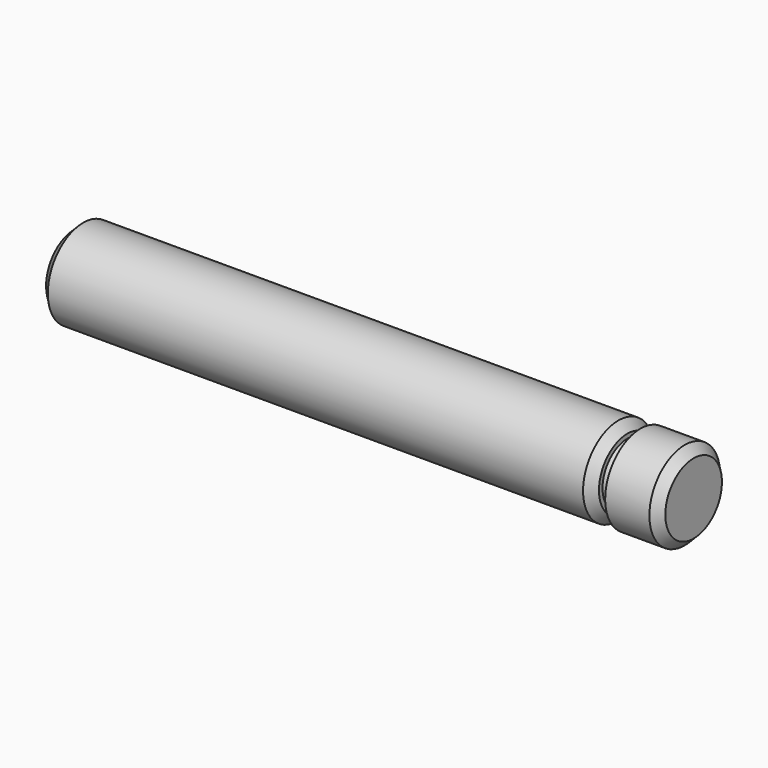
from build123d import *

# Parameters (mm, degrees)
F2_SIZE = 1


with BuildPart() as f1:
    # F0 (on Front) → F1 (revolve)
    with BuildSketch(Plane.XZ):
        Polygon((-83.1480100751, 5), (-83.1480100751, 0), (-74.9320751429, 0), (-13.1480100751, 0), (-13.1480100751, 5), (-19.1480100751, 5), (-19.1480100751, 3.5), (-20.6480100751, 3.5), (-20.6480100751, 5), (-74.9320751429, 5), align=None)
    revolve(axis=Axis((-48.1480100751, 0, 0), (1, 0, 0)))

    # F2
    f2_edges = [f1.edges().sort_by_distance(p)[0] for p in [
        (-13.14801, 0, -5),
        (-20.64801, 0, -5),
        (-83.14801, 0, -5),
    ]]
    chamfer(f2_edges, length=F2_SIZE)


solid = f1.part
